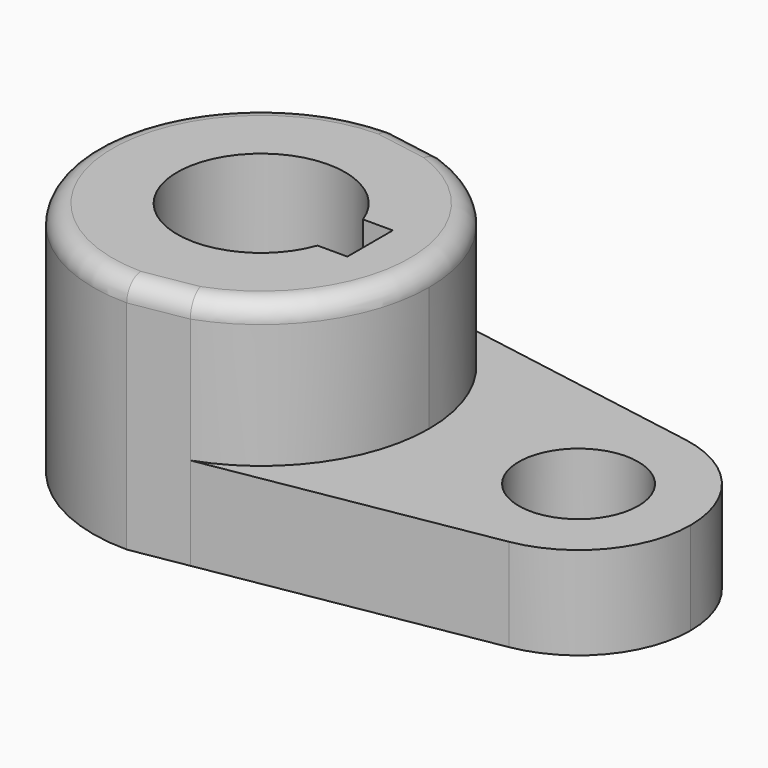
from build123d import *

# Parameters (mm, degrees)
F1_DEPTH    = 40.2336
F0_R        = 10.16
F2_DEPTH    = 15.7734
F3_T1_DEPTH = 37.7177817865
F3_T3_DEPTH = 37.7177817865
F3_T6_ANGLE = 213.1574660215
F3_T8_ANGLE = 174.2489977384


# Not quite as in the source:
# - a fillet or chamfer that OpenCascade refuses, or shapes differently, is made with other operations: its cross-section is extruded or revolved along the edge and cut away or added


with BuildPart() as f1:
    # F0 (on Top) → F1 (new body)
    with BuildSketch(Plane.XY):
        with BuildLine():
            Line((-19.1519816242, 26.9452959039), (-28.6641661078, 28.575))
            ThreePointArc((-28.6641661078, 28.575), (-57.2391661078, 0), (-28.6641661078, -28.575))
            Line((-28.6641661078, -28.575), (-19.1519816242, -26.9452959039))
            ThreePointArc((-19.1519816242, -26.9452959039), (-5.3367005723, -16.5033322905), (-0.0891661078, 0))
            ThreePointArc((-0.0891661078, 0), (-5.3367005723, 16.5033322905), (-19.1519816242, 26.9452959039))
        make_face()
        with BuildLine():
            ThreePointArc((-15.2164012284, -4.826), (-42.9516661078, 0), (-15.2164012284, 4.826))
            Line((-15.2164012284, 4.826), (-10.1348661078, 4.826))
            Line((-10.1348661078, 4.826), (-10.1348661078, -4.826))
            Line((-10.1348661078, -4.826), (-15.2164012284, -4.826))
        make_face(mode=Mode.SUBTRACT)
    extrude(amount=F1_DEPTH)

    # F0 (on Top) → F2 (join)
    with BuildSketch(Plane.XY):
        with BuildLine():
            Line((28.5277611544, 18.7764181619), (-19.1519816242, 26.9452959039))
            ThreePointArc((-19.1519816242, 26.9452959039), (-5.3367005723, 16.5033322905), (-0.0891661078, 0))
            ThreePointArc((-0.0891661078, 0), (-5.3367005723, -16.5033322905), (-19.1519816242, -26.9452959039))
            Line((-19.1519816242, -26.9452959039), (28.5277611544, -18.7764181619))
            ThreePointArc((28.5277611544, -18.7764181619), (6.2608338922, 0), (28.5277611544, 18.7764181619))
        make_face()
        with BuildLine():
            ThreePointArc((44.3608338922, 0), (39.8742291753, 12.2804730295), (28.5277611544, 18.7764181619))
            ThreePointArc((28.5277611544, 18.7764181619), (6.2608338922, 0), (28.5277611544, -18.7764181619))
            ThreePointArc((28.5277611544, -18.7764181619), (39.8742291753, -12.2804730295), (44.3608338922, 0))
        make_face()
        with Locations((25.3108338922, 0)):
            Circle(F0_R, mode=Mode.SUBTRACT)
    extrude(amount=F2_DEPTH)

    # F3: fillet of radius 3.302 on 4 edges, made by hand

    # F3_s2 → F3_t1 (cut)
    with BuildSketch(Plane(origin=(-46.4348249971, -7.955588396, 0), x_dir=(0, 0, 1), z_dir=(0.9856387487, 0.1688675728, 0))):
        with BuildLine():
            ThreePointArc((36.9316, 23.3241790854), (39.2664665915, 22.3570456768), (40.2336, 20.0221790854))
            Line((40.2336, 20.0221790854), (40.2336, 23.3241790854))
            Line((40.2336, 23.3241790854), (36.9316, 23.3241790854))
        make_face()
    extrude(amount=F3_T1_DEPTH, mode=Mode.SUBTRACT)

    # F3_s4 → F3_t3 (cut)
    with BuildSketch(Plane(origin=(-9.258717755, 1.5862781337, 0), x_dir=(0, 0, 1), z_dir=(-0.9856387487, 0.1688675728, 0))):
        with BuildLine():
            ThreePointArc((36.9316, 23.3241790854), (39.2664665915, 22.3570456768), (40.2336, 20.0221790854))
            Line((40.2336, 20.0221790854), (40.2336, 23.3241790854))
            Line((40.2336, 23.3241790854), (36.9316, 23.3241790854))
        make_face()
    extrude(amount=F3_T3_DEPTH, mode=Mode.SUBTRACT)

    # F3_s5 → F3_t6 (revolve, cut)
    with BuildSketch(Plane(origin=(-26.3304812045, 7.8388166507, 0), x_dir=(0, 0, 1), z_dir=(0.95842855, -0.2853326385, 0))):
        with BuildLine():
            ThreePointArc((36.9316, -20.3961778531), (39.2664665915, -19.4290444446), (40.2336, -17.0941778531))
            Line((40.2336, -17.0941778531), (40.2336, -20.3961778531))
            Line((40.2336, -20.3961778531), (36.9316, -20.3961778531))
        make_face()
    revolve(axis=Axis((-28.6641661078, 0, 40.2336), (0, 0, 1)), revolution_arc=F3_T6_ANGLE, mode=Mode.SUBTRACT)

    # F3_s7 → F3_t8 (revolve, cut)
    with BuildSketch(Plane(origin=(-28.5920293734, 1.4361530661, 0), x_dir=(0, 0, 1), z_dir=(-0.9987408987, 0.0501658971, 0))):
        with BuildLine():
            ThreePointArc((40.2336, 23.835036392), (39.2664665915, 26.1699029835), (36.9316, 27.137036392))
            Line((36.9316, 27.137036392), (40.2336, 27.137036392))
            Line((40.2336, 27.137036392), (40.2336, 23.835036392))
        make_face()
    revolve(axis=Axis((-28.6641661078, 0, 40.2336), (0, 0, -1)), revolution_arc=F3_T8_ANGLE, mode=Mode.SUBTRACT)


solid = f1.part
